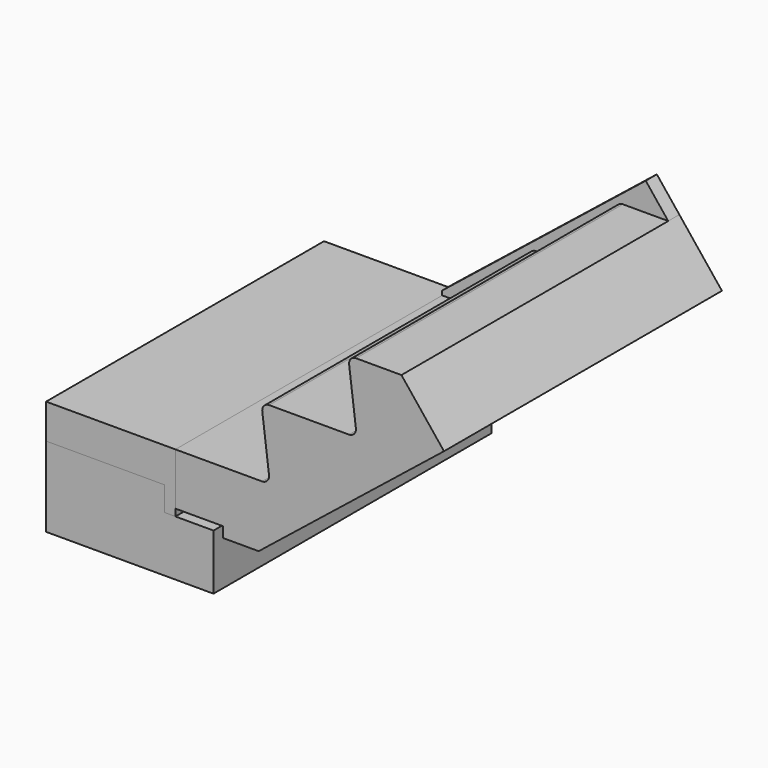
from build123d import *

# Parameters (mm, degrees)
F0_W     = 481.9511
F0_H     = 50
F1_DEPTH = 1000
F2_DEPTH = 1000
F3_DEPTH = 1000
F4_DEPTH = 40


# Not quite as in the source:
# - ends of sketch curves that miss each other by under 0.0002 mm in the source are joined


with BuildPart() as f1:
    # F0 (on Front) → F1 (new body)
    with BuildSketch(Plane.XZ):
        Polygon((-90.785567, -193.770768), (-200.376776, -193.770768), (-232.113212, -193.770768), (-232.113212, -123.770768), (-572.736667, -123.770768), (-572.736667, -303.770768), (-90.785567, -303.770768), align=None)
        with Locations((-331.761117, -328.770768)):
            Rectangle(F0_W, F0_H)
    extrude(amount=F1_DEPTH)


with BuildPart() as f2:
    # F0 (on Front) → F2 (new body)
    with BuildSketch(Plane.XZ):
        Polygon((-200.376776, -173.770768), (-200.376776, -23.770768), (-572.736667, -23.770768), (-572.736667, -123.770768), (-232.113212, -123.770768), (-232.113212, -193.770768), (-200.376776, -193.770768), align=None)
    extrude(amount=F2_DEPTH)


with BuildPart() as f3:
    # F0 (on Front) → F3 (new body)
    with BuildSketch(Plane.XZ):
        with BuildLine():
            Line((49.157493, -23.770768), (-200.376776, -23.770768))
            Line((-200.376776, -23.770768), (-200.376776, -173.770768))
            Line((-200.376776, -173.770768), (-90.785567, -173.770768))
            Line((-90.785567, -173.770768), (-63.950427, -173.770768))
            Line((-63.950427, -173.770768), (-63.950427, -203.770768))
            Line((-63.950427, -203.770768), (39.214433, -203.770768))
            Line((39.214433, -203.770768), (226.7144330686, -53.7707680857))
            Line((226.7144330686, -53.7707680857), (572.661266, 222.986698))
            Line((572.661266, 222.986698), (450.1545409622, 376.2292319698))
            Line((450.1545409622, 376.2292319698), (319.468781, 376.229232))
            ThreePointArc((319.468781, 376.229232), (304.4752173606, 369.4652831252), (299.6232235119, 353.748536939))
            Line((299.6232235119, 353.748536939), (319.00305, 198.709926))
            ThreePointArc((319.00305, 198.709926), (314.1510563111, 182.9931805028), (299.157493, 176.229232))
            Line((299.157493, 176.229232), (69.468781, 176.229232))
            ThreePointArc((69.468781, 176.229232), (54.4752173606, 169.4652831252), (49.6232235119, 153.748536939))
            Line((49.6232235119, 153.748536939), (69.00305, -1.290074))
            ThreePointArc((69.00305, -1.290074), (64.1510563111, -17.0068194972), (49.157493, -23.770768))
        make_face()
    extrude(amount=F3_DEPTH)


with BuildPart() as f4:
    # F0 (on Front) → F4 (new body)
    with BuildSketch(Plane.XZ):
        with BuildLine():
            Line((-200.376776, -11.256305), (-200.376776, -23.770768))
            Line((-200.376776, -23.770768), (49.157493, -23.770768))
            ThreePointArc((49.157493, -23.770768), (64.1510563111, -17.0068194972), (69.0030506112, -1.2900739236))
            Line((69.0030506112, -1.2900739236), (49.623224, 153.748537))
            ThreePointArc((49.623224, 153.748537), (54.4752173606, 169.4652831252), (69.468781, 176.229232))
            Line((69.468781, 176.229232), (299.157493, 176.229232))
            ThreePointArc((299.157493, 176.229232), (314.1510563111, 182.9931805028), (319.0030506112, 198.7099260764))
            Line((319.0030506112, 198.7099260764), (299.623224, 353.748537))
            ThreePointArc((299.623224, 353.748537), (304.4752173606, 369.4652831252), (319.468781, 376.229232))
            Line((319.468781, 376.229232), (450.154541, 376.229232))
            Line((450.154541, 376.229232), (385.3341629587, 457.312445967))
            Line((385.3341629587, 457.312445967), (-200.376776, -11.256305))
        make_face()
    extrude(amount=F4_DEPTH)


solid = Compound([f1.part, f2.part, f3.part, f4.part])
